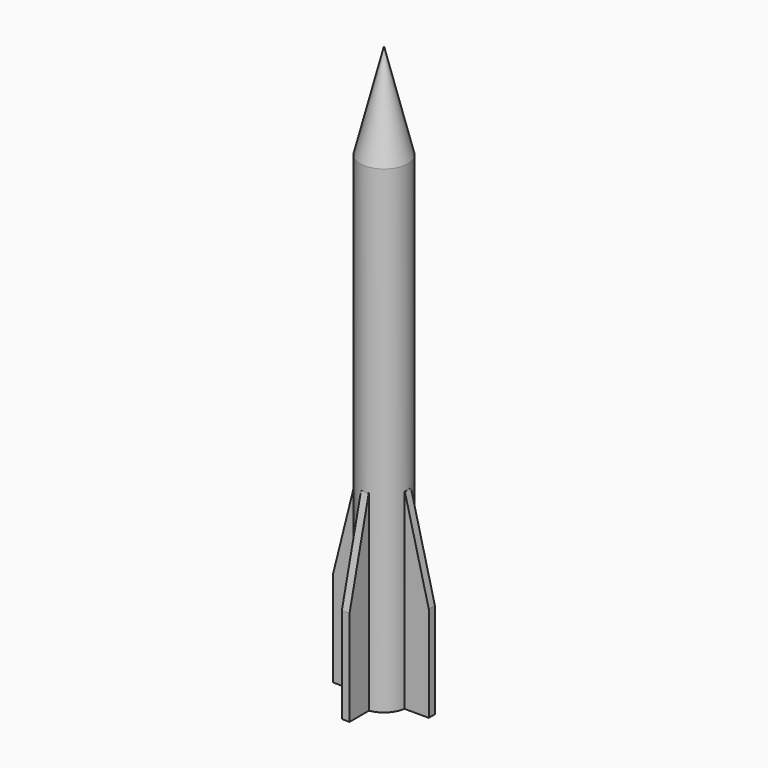
from build123d import *

# Parameters (mm, degrees)
F3_DEPTH   = 25.4
F4_SIZE2   = 12.69999
F4_SIZE    = 3.17499
F4_2_SIZE2 = 12.69999
F4_2_SIZE  = 3.17499
F5_SIZE2   = 12.69999
F5_SIZE    = 3.17499
F5_2_SIZE2 = 12.69999
F5_2_SIZE  = 3.17499


# Not quite as in the source:
# - a fillet or chamfer is up to 0.001 mm smaller than in the source, because OpenCascade refuses the exact size


with BuildPart() as f2:
    # F1 (on Front) → F2 (revolve)
    with BuildSketch(Plane.XZ):
        Polygon((0, 76.2), (0, 0), (3.175, 0), (3.175, 63.5), align=None)
    revolve(axis=Axis((0, 0, 38.1), (0, 0, 1)))

    # F0 (on Top) → F3 (join)
    with BuildSketch(Plane.XY):
        with BuildLine():
            ThreePointArc((3.1340965205, 0.508), (3.1647576094, 0.2548220431), (3.175, 0))
            ThreePointArc((3.175, 0), (3.1647576094, -0.2548220431), (3.1340965205, -0.508))
            Line((3.1340965205, -0.508), (6.35, -0.508))
            Line((6.35, -0.508), (6.35, 0.508))
            Line((6.35, 0.508), (3.1340965205, 0.508))
        make_face()
        with BuildLine():
            Line((0.508, -6.35), (0.508, -3.1340965205))
            ThreePointArc((0.508, -3.1340965205), (0, -3.175), (-0.508, -3.1340965205))
            Line((-0.508, -3.1340965205), (-0.508, -6.35))
            Line((-0.508, -6.35), (0.508, -6.35))
        make_face()
        with BuildLine():
            ThreePointArc((-3.1340965205, -0.508), (-3.175, 0), (-3.1340965205, 0.508))
            Line((-3.1340965205, 0.508), (-6.35, 0.508))
            Line((-6.35, 0.508), (-6.35, -0.508))
            Line((-6.35, -0.508), (-3.1340965205, -0.508))
        make_face()
        with BuildLine():
            ThreePointArc((-0.508, 3.1340965205), (0, 3.175), (0.508, 3.1340965205))
            Line((0.508, 3.1340965205), (0.508, 6.35))
            Line((0.508, 6.35), (-0.508, 6.35))
            Line((-0.508, 6.35), (-0.508, 3.1340965205))
        make_face()
    extrude(amount=F3_DEPTH)

    # F4 (size 3.175 and 12.7 in the source; OpenCascade refuses exactly that, so slightly less here)
    f4_edges = [f2.edges().sort_by_distance(p)[0] for p in [
        (0, -6.35, 25.4),
    ]]
    f4_side = f2.faces().sort_by_distance((0, -4.755677, 25.4))[0]
    chamfer(f4_edges, length=F4_SIZE, length2=F4_SIZE2, reference=f4_side)

    # F4#2 (size 3.175 and 12.7 in the source; OpenCascade refuses exactly that, so slightly less here)
    f4_2_edges = [f2.edges().sort_by_distance(p)[0] for p in [
        (6.35, 0, 25.4),
    ]]
    f4_2_side = f2.faces().sort_by_distance((4.755677, 0, 25.4))[0]
    chamfer(f4_2_edges, length=F4_2_SIZE, length2=F4_2_SIZE2, reference=f4_2_side)

    # F5 (size 3.175 and 12.7 in the source; OpenCascade refuses exactly that, so slightly less here)
    f5_edges = [f2.edges().sort_by_distance(p)[0] for p in [
        (-6.35, 0, 25.4),
    ]]
    f5_side = f2.faces().sort_by_distance((-4.755677, 0, 25.4))[0]
    chamfer(f5_edges, length=F5_SIZE, length2=F5_SIZE2, reference=f5_side)

    # F5#2 (size 3.175 and 12.7 in the source; OpenCascade refuses exactly that, so slightly less here)
    f5_2_edges = [f2.edges().sort_by_distance(p)[0] for p in [
        (0, 6.35, 25.4),
    ]]
    f5_2_side = f2.faces().sort_by_distance((0, 4.755677, 25.4))[0]
    chamfer(f5_2_edges, length=F5_2_SIZE, length2=F5_2_SIZE2, reference=f5_2_side)


solid = f2.part
